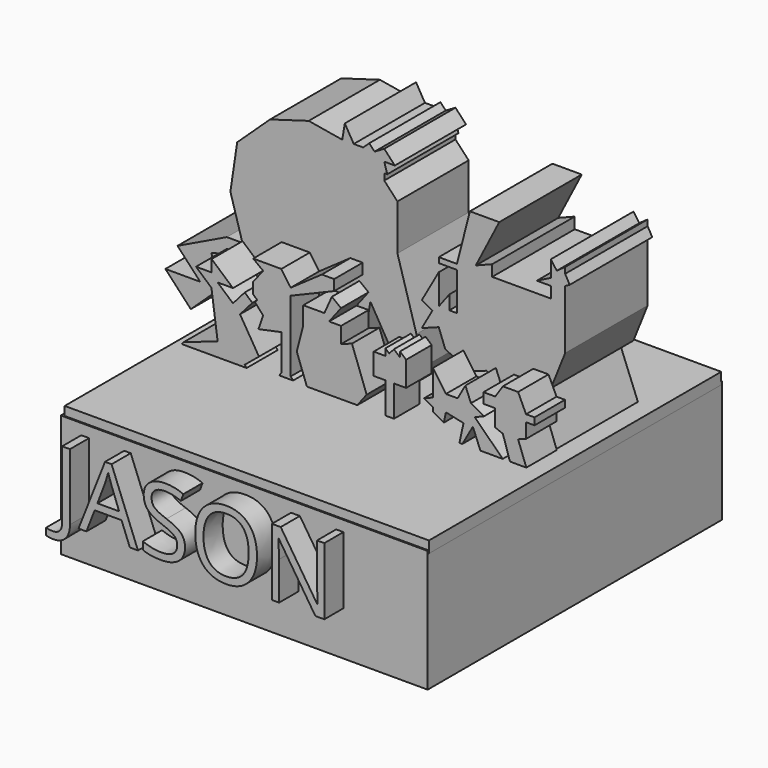
from build123d import *

# Parameters (mm, degrees)
F0_W           = 151.7640277743
F0_H           = 50.5070704967
F1_DEPTH       = 75.692
F1_DEPTH_BACK  = 76.454
F3_START       = -5.334
F3_DEPTH       = 36.83
F5_DEPTH       = 42.672
F7_DEPTH       = 15.748
F9_DEPTH       = 15.748
F11_START      = 2.54
F11_DEPTH      = 13.208
F13_START      = 1.524
F13_DEPTH      = 14.224
F15_START      = 0.508
F15_DEPTH      = 14.732
F17_START      = 1.778
F17_DEPTH      = 16.002
F18_TEXT_SIZE  = 38.8633873728
F19_DEPTH      = 85.598
F20_W          = 79.5727889054
F20_H          = 4.7495681792
F20_W_2        = 71.1200018413
F21_DEPTH      = 75.946
F21_DEPTH_BACK = 75.184


# Not quite as in the source:
# - Text() gives the source's letters only with a copy of the font that has no kerning and outlines rounded to 1/6400 em; it was checked with that copy


with BuildPart() as f1:
    # F0 (on Front) → F1 (new body, two sides)
    with BuildSketch(Plane.XZ) as f1_sk:
        with Locations((0.1214109361, -50.6284823641)):
            Rectangle(F0_W, F0_H)
    extrude(amount=F1_DEPTH)
    extrude(f1_sk.sketch, amount=-F1_DEPTH_BACK)

    # F18 (on Front) → F19 (join)
    with BuildSketch(Plane.XZ):
        with Locations((-70.8911567926, -57.5663931668)):
            Text('JASON', F18_TEXT_SIZE, font='Open Sans', text_align=(TextAlign.LEFT, TextAlign.BOTTOM))
    extrude(amount=F19_DEPTH)


with BuildPart() as f3:
    # F2 (on Front) → F3 (new body)
    with BuildSketch(Plane.XZ.offset(F3_START)):
        Polygon((-59.8501488566, -21.4897878468), (-59.8501488566, -23.9180140197), (-40.9328403471, -23.9180140197), (-40.9328403471, -17.9666938573), (-39.5242605419, -9.631286444), (-26.3246274011, -1.926445355), (-28.8667935634, -16.9699598199), (-38.0434047872, -15.4192270711), (-38.0434047872, -23.9180140197), (-17.2011012221, -23.9180140197), (-12.5232289252, 3.7637483329), (-1.3258133965, -15.4192270711), (-10.800011456, -15.4192270711), (-10.800011456, -23.9180140197), (3.0151365754, -23.9180140197), (6.5288132535, -15.4192270711), (6.5288132535, -1.926445355), (-1.3258133965, 24.9089510924), (-1.3258133965, 43.8294559717), (-6.7793508673, 49.6571958065), (-6.7793508673, 52.3436654009), (-5.546891752, 52.3436654009), (-6.7793508673, 56.5543720887), (-2.4026648759, 56.5543720887), (-6.7793508673, 61.2313707218), (-10.800011456, 58.8844455779), (-12.9962392521, 61.2313707218), (-15.5042020605, 58.8844455779), (-19.4124838058, 58.8844455779), (-23.0904626915, 65.1854155043), (-24.1552479565, 58.8844455779), (-38.0434047872, 61.2313707218), (-54.0224090219, 56.5543720887), (-67.6204636693, 43.8294559717), (-70.4266597213, 24.9089510924), (-65.4457787651, 7.8917304054), (-71.8936855621, 7.8917304054), (-92.3080195735, -1.926445355), (-82.9182863235, -11.9604687374), (-97.311494559, -11.9604687374), (-86.8034437299, -23.1895446777), (-74.8038684971, -11.9604687374), (-78.3046558499, 0), (-65.4457787651, 3.7637483329), (-71.8936855621, 0), (-65.4457787651, 0), (-65.4457787651, -4.4527893136), (-54.0224090219, -15.4192270711), align=None)
    extrude(amount=-F3_DEPTH)


with BuildPart() as f5:
    # F4 (on Front) → F5 (new body)
    with BuildSketch(Plane.XZ):
        Polygon((45.0491532683, -4.7350381501), (45.0491532683, -25.1321252435), (68.8457563519, -23.1639934637), (60.5897903442, -2.3068133742), (66.417530179, 0), (72.3141783793, 14.7212772829), (72.3141783793, 32.6596200466), (72.3141783793, 39.1544317686), (74.1878449917, 40.1871167123), (72.3141783793, 43.5866303742), (72.3141783793, 46.0640768513), (68.8457563519, 43.5866303742), (66.417530179, 46.9861440361), (66.417530179, 40.1871167123), (60.5897903442, 37.2732467949), (66.417530179, 37.2732467949), (66.417530179, 32.6596200466), (42.1352833509, 32.6596200466), (42.1352833509, 37.2732467949), (35.3362560272, 34.6022024751), (45.0491532683, 53.5423532128), (32.9080335796, 53.5423532128), (27.565933764, 32.6596200466), (20.0384408236, 32.6596200466), (20.0384408236, 30.4742194712), (27.565933764, 30.4742194712), (27.565933764, 14.7212772829), (24.409243837, 14.7212772829), (24.409243837, 20.5184984952), (20.0384408236, 14.7212772829), (20.0384408236, 27.1739801626), (13.0106757645, 14.7212772829), (17.3673927784, 12.2625352815), (13.0106757645, 4.5427407168), (20.0384408236, 7.1632624604), (22.7094870061, 0), (32.9080335796, -4.7350381501), (39.7070609033, -2.3068133742), align=None)
    extrude(amount=-F5_DEPTH)


with BuildPart() as f7:
    # F6 (on Front) → F7 (new body)
    with BuildSketch(Plane.XZ):
        Polygon((63.2608383894, -25.3749471158), (70.3026875854, -25.617768988), (65.4462426901, -12.5053562224), (68.7441113363, -11.2839244662), (68.7441113363, -5.2206832916), (72.2452700138, -5.2206832916), (72.2452700138, -2.3068133742), (68.7441113363, -2.3068133742), (65.4462426901, 4.7350381501), (59.1328553855, 4.7350381501), (55.9761673212, 0), (51.1197187006, 0), (51.1197187006, -4.2493930086), (55.9761673212, -4.2493930086), (55.9761673212, -11.2839244662), (59.1328553855, -12.5053562224), align=None)
    extrude(amount=F7_DEPTH)


with BuildPart() as f9:
    # F8 (on Front) → F9 (new body)
    with BuildSketch(Plane.XZ):
        Polygon((46.7489100993, -13.9622911811), (51.6053624451, -26.1034145951), (62.5323727727, -25.1321252435), (47.5299740155, -10.2464862709), (51.3046512807, -8.7366144383), (45.9433744602, -5.7063279673), (43.6608418725, 0), (40.43552652, -5.7063279673), (35.5852137376, -5.7063279673), (30.2735996622, 2.0639908034), (30.2735996622, -8.7366144383), (26.498922397, -10.2464862709), (30.2735996622, -12.3799992067), (30.2735996622, -13.9622911811), (34.697640139, -16.4628354456), (35.5852137376, -12.3799992067), (42.8637526929, -13.9622911811), (40.43552652, -25.1321252435), align=None)
    extrude(amount=F9_DEPTH)


with BuildPart() as f11:
    # F10 (on Front) → F11 (new body)
    with BuildSketch(Plane.XZ.offset(F11_START)):
        Polygon((5.7119159028, -21.9754315913), (5.7119159028, -25.3749471158), (18.8243277371, -24.6464796364), (19.1178435109, -21.9754315913), (14.1072242852, -21.9754315913), (14.1072242852, -8.863019757), (19.1178435109, -8.863019757), (19.1178435109, 1.3962291414), (16.6125338981, 3.6124633883), (16.6125338981, 1.3962291414), (14.1072242852, 3.6124633883), (12.1467104182, 1.3962291414), (10.568363592, 2.7924582828), (10.568363592, 0), (5.7119159028, 0), (5.7119159028, -8.863019757), (10.568363592, -8.863019757), (10.568363592, -21.9754315913), align=None)
    extrude(amount=F11_DEPTH)


with BuildPart() as f13:
    # F12 (on Front) → F13 (new body)
    with BuildSketch(Plane.XZ.offset(F13_START)):
        Polygon((-20.755732432, -24.8893015087), (-3.5153380595, -24.8893015087), (2.7980469167, -16.6333392262), (-3.2725157216, 0), (-7.7943062975, -1.6502887698), (-7.7943062975, 4.977860488), (-12.7425920218, 4.977860488), (-7.7943062975, 11.4486935603), (-11.5888054075, 14.3503702945), (-14.685170725, 7.4060852639), (-23.4267804772, 7.4060852639), (-23.4267804772, 0), (-26.0978266597, -10.3199547157), align=None)
    extrude(amount=F13_DEPTH)


with BuildPart() as f15:
    # F14 (on Front) → F15 (new body)
    with BuildSketch(Plane.XZ.offset(F15_START)):
        Polygon((-36.2963713706, -25.1321252435), (-25.8550047874, -24.4036559016), (-29.0116965771, -20.5184984952), (-29.0116965771, 8.863019757), (-11.0428333282, 16.3905154914), (-11.0428333282, 20.7613185048), (-16.1421056837, 20.7613185048), (-29.0116965771, 11.7768896744), (-32.8968539834, 17.3421167266), (-37.9961282015, 17.3421167266), (-44.552333653, 17.3421167266), (-40.4243506491, 14.2051139846), (-44.552333653, 8.863019757), (-44.552333653, 2.5496359449), (-40.4243506491, -2.0639908034), (-42.3669330776, -7.6489071362), (-32.8968539834, -5.6684176043), (-32.8968539834, -20.5184984952), align=None)
    extrude(amount=F15_DEPTH)


with BuildPart() as f17:
    # F16 (on Front) → F17 (new body)
    with BuildSketch(Plane.XZ.offset(F17_START)):
        Polygon((-57.2175836053, -24.6464796364), (-42.6097549498, -24.8893015087), (-46.0092686117, -20.7613185048), (-40.1109365184, -15.9038710506), (-47.9518473148, -3.0352806207), (-42.852576822, 2.7924582828), (-46.0092686117, 5.5545630312), (-50.8695102653, 0), (-57.2175836053, 5.5545630312), (-50.8695102653, 5.5545630312), (-59.6927772003, 13.274920013), (-59.6927772003, 8.3773750812), (-66.1635324359, 8.3773750812), (-59.7807690691, 2.7924582828), (-57.2175836053, -15.9038710506), (-51.6662139456, -20.7613185048), align=None)
        Polygon((-74.8747910402, -24.8893015087), (-57.2175836053, -24.6464796364), (-51.6662139456, -20.7613185048), (-57.2175836053, -15.9038710506), (-71.262806654, -20.7613185048), align=None)
    extrude(amount=F17_DEPTH)


with BuildPart() as f21:
    # F20 (on Front) → F21 (new body, two sides)
    with BuildSketch(Plane.XZ) as f21_sk:
        with Locations((-34.7774813417, -24.0897005424)):
            Rectangle(F20_W, F20_H)
        with Locations((40.5689140316, -24.0897005424)):
            Rectangle(F20_W_2, F20_H)
    extrude(amount=-F21_DEPTH)
    extrude(f21_sk.sketch, amount=F21_DEPTH_BACK)


solid = Compound([f1.part, f3.part, f5.part, f7.part, f9.part, f11.part, f13.part, f15.part, f17.part, f21.part])
